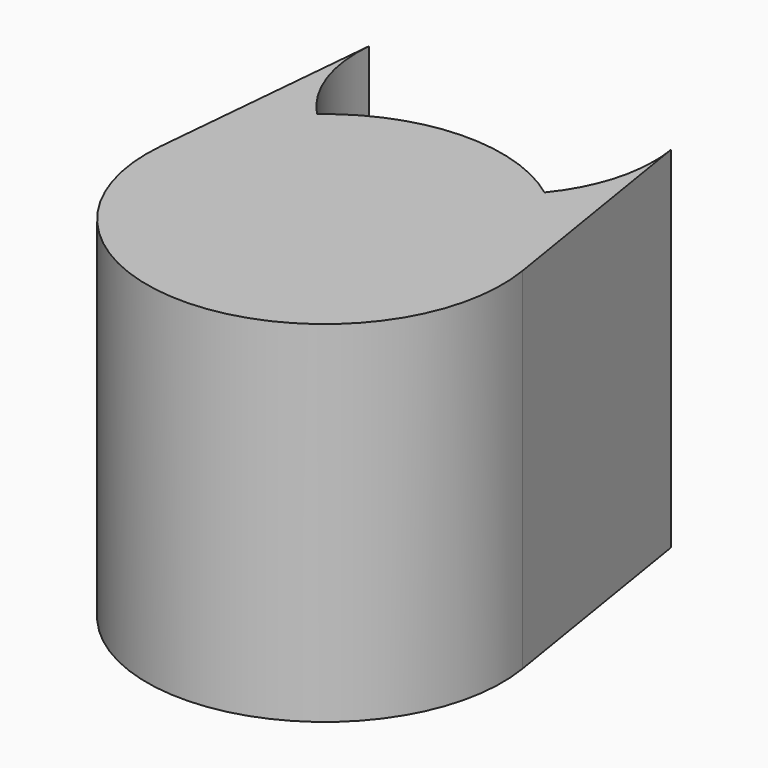
from build123d import *

# Parameters (mm, degrees)
F1_DEPTH = 901.7


# Not quite as in the source:
# - a feature names something its author has since deleted; it is built from what else it names


with BuildPart() as f1:
    # F0 (on Top) → F1 (new body)
    with BuildSketch(Plane.XY):
        with BuildLine():
            ThreePointArc((-297.3647676133, -1105.7196050937), (-380.9510446566, -968.4252745053), (-400.480099263, -808.8789961161))
            Line((-400.480099263, -808.8789961161), (-455.3190686334, -1411.5741151153))
            ThreePointArc((-455.3190686334, -1411.5741151153), (-406.2265189052, -1243.2133743356), (-297.3647676132, -1105.7196050937))
        make_face()
        with BuildLine():
            ThreePointArc((-297.3647676133, -1105.7196050937), (-7.9006621425, -1224.1765088207), (272.7039865955, -1086.0369507529))
            ThreePointArc((272.7039865955, -1086.0369507529), (-15.7762559112, -996.0756718787), (-297.3647676132, -1105.7196050937))
        make_face()
        with BuildLine():
            ThreePointArc((355.1002524449, -782.7912184935), (358.7374692929, -813.000356121), (359.9524579315, -843.4034011198))
            ThreePointArc((359.9524579315, -843.4034011198), (337.477444802, -972.3252138184), (272.7039865955, -1086.0369507529))
            ThreePointArc((272.7039865955, -1086.0369507529), (390.7896356908, -1215.6949507084), (451.377353416, -1380.2687819682))
            Line((451.377353416, -1380.2687819682), (355.1002524449, -782.7912184935))
        make_face()
        with BuildLine():
            ThreePointArc((451.377353416, -1380.2687819682), (390.7896356908, -1215.6949507084), (272.7039865955, -1086.0369507529))
            ThreePointArc((272.7039865955, -1086.0369507529), (-7.9006621425, -1224.1765088207), (-297.3647676133, -1105.7196050937))
            ThreePointArc((-297.3647676132, -1105.7196050937), (-406.2265189052, -1243.2133743356), (-455.3190686334, -1411.5741151153))
            ThreePointArc((-455.3190686334, -1411.5741151153), (-20.7359810574, -1909.7329262105), (457.2, -1453.0034011198))
            ThreePointArc((457.2, -1453.0034011198), (455.7420136337, -1416.5197471212), (451.377353416, -1380.2687819682))
        make_face()
    extrude(amount=F1_DEPTH)


solid = f1.part
